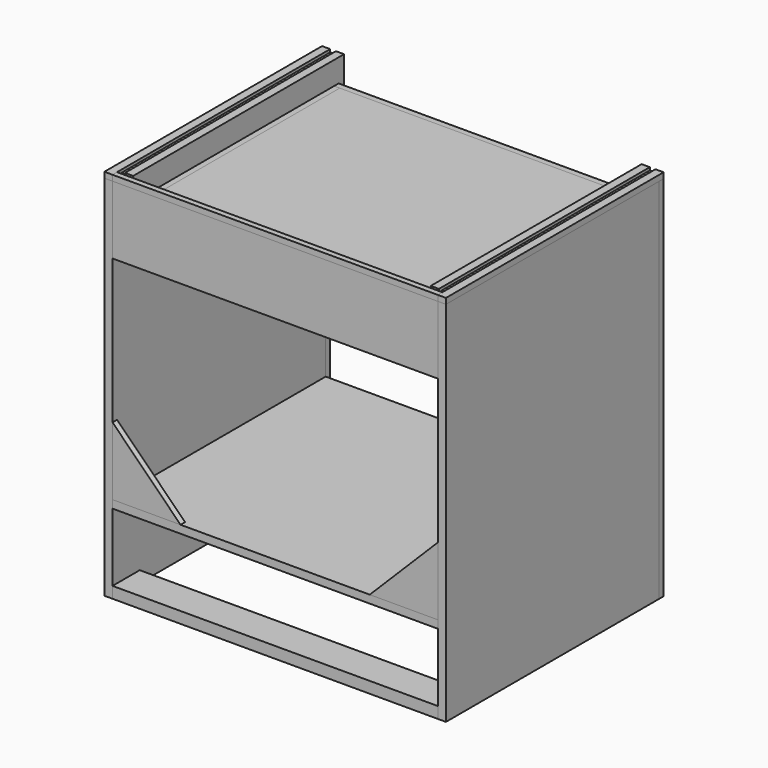
from build123d import *

# Parameters (mm, degrees)
F0_W           = 584.2
F0_H           = 208.915
F0_W_2         = 25.4
F0_W_3         = 635
F0_H_2         = 26.67
F1_DEPTH       = 18.25625
F2_DEPTH       = 4.1402
F3_DEPTH       = 18.25625
F4_DEPTH       = 18.25625
F9_DEPTH       = 54.76875
F8_W           = 12.7
F8_H           = 546.1
F10_DEPTH      = 54.76875
F12_DEPTH      = 660.401
F16_DEPTH      = 304.8
F16_DEPTH_BACK = 285.75
F15_W          = 12.7
F15_H          = 35.56
F17_DEPTH      = 304.8
F17_DEPTH_BACK = 279.4
F18_DEPTH      = 694.53225
F18_DEPTH_BACK = 34.13225
F19_W          = 18.25625
F19_H          = 12.7
F20_DEPTH      = 304.8
F19_H_2        = 823.515625
F21_DEPTH      = 304.8
F21_DEPTH_BACK = 292.1
F22_W          = 18.25625
F22_H          = 12.7
F23_DEPTH      = 823.515625
F24_W          = 76.2
F24_H          = 25.4
F25_DEPTH      = 728.6625
F24_W_2        = 596.9
F24_H_2        = 17.6944031715
F26_W          = 12.7
F26_H          = 152.4
F27_DEPTH      = 728.6625
F26_H_2        = 12.7
F28_DEPTH      = 728.6625
F30_DEPTH      = 12.7
F32_DEPTH      = 703.2625


# Not quite as in the source:
# - an extrude ends at something that could not be found from the text; its depth is read off the source's solid
# - a feature of the source that left no trace in its solid (it failed there, or was rolled back) is left out
# - a pattern or mirror of a feature is missing from the dataset's text; its kind, count and spacing are read off the source's solid


with BuildPart() as f1:
    # F0 (on Top) → F1 (new body)
    with BuildSketch(Plane.XY):
        Polygon((317.5, 241.3), (-317.5, 241.3), (-317.5, 215.9), (-292.1, 215.9), (292.1, 215.9), (317.5, 215.9), align=None)
        with Locations((0, 111.4425)):
            Rectangle(F0_W, F0_H)
        with Locations((-304.8, 111.4425)):
            Rectangle(F0_W_2, F0_H)
        with Locations((304.8, 111.4425)):
            Rectangle(F0_W_2, F0_H)
        Polygon((-292.1, 6.985), (-317.5, 6.985), (-317.5, -18.415), (317.5, -18.415), (317.5, 6.985), (292.1, 6.985), align=None)
        with Locations((0, -31.75)):
            Rectangle(F0_W_3, F0_H_2)
        Polygon((317.5, -45.085), (-317.5, -45.085), (-317.5, -70.485), (-292.1, -70.485), (292.1, -70.485), (317.5, -70.485), align=None)
        with Locations((304.8, -174.9425)):
            Rectangle(F0_W_2, F0_H)
        with Locations((0, -174.9425)):
            Rectangle(F0_W, F0_H)
        Polygon((-292.1, -279.4), (-317.5, -279.4), (-317.5, -304.8), (317.5, -304.8), (317.5, -279.4), (292.1, -279.4), align=None)
        with Locations((-304.8, -174.9425)):
            Rectangle(F0_W_2, F0_H)
    extrude(amount=F1_DEPTH)


with BuildPart() as f1_copies_1:
    # F1_copies: instance of F1
    add(f1.part.mirror(Plane(origin=(0, 0, -9.128125), x_dir=(-1, 0, 0), z_dir=(0, 0, -1))))


with BuildPart() as f1_1:
    add(f1.part)

    # F0 (on Top) → F2 (cut)
    with BuildSketch(Plane.XY):
        with Locations((0, -31.75)):
            Rectangle(F0_W_3, F0_H_2)
    extrude(amount=F2_DEPTH, mode=Mode.SUBTRACT)


with BuildPart() as f3:
    # F0 (on Top) → F3 (new body)
    with BuildSketch(Plane.XY):
        Polygon((317.5, -45.085), (-317.5, -45.085), (-317.5, -70.485), (-292.1, -70.485), (292.1, -70.485), (317.5, -70.485), align=None)
    extrude(amount=-F3_DEPTH)


with BuildPart() as f3b:
    # F0 (on Top) → F3, piece 2 (new body)
    with BuildSketch(Plane.XY):
        Polygon((-292.1, 6.985), (-317.5, 6.985), (-317.5, -18.415), (317.5, -18.415), (317.5, 6.985), (292.1, 6.985), align=None)
    extrude(amount=-F3_DEPTH)


with BuildPart() as f3c:
    # F0 (on Top) → F3, piece 3 (new body)
    with BuildSketch(Plane.XY):
        Polygon((317.5, 241.3), (-317.5, 241.3), (-317.5, 215.9), (-292.1, 215.9), (292.1, 215.9), (317.5, 215.9), align=None)
    extrude(amount=-F3_DEPTH)


with BuildPart() as f3d:
    # F0 (on Top) → F3, piece 4 (new body)
    with BuildSketch(Plane.XY):
        Polygon((-292.1, -279.4), (-317.5, -279.4), (-317.5, -304.8), (317.5, -304.8), (317.5, -279.4), (292.1, -279.4), align=None)
    extrude(amount=-F3_DEPTH)


with BuildPart() as f4:
    # F0 (on Top) → F4 (new body)
    with BuildSketch(Plane.XY):
        with Locations((304.8, -174.9425)):
            Rectangle(F0_W_2, F0_H)
    extrude(amount=-F4_DEPTH)


with BuildPart() as f4b:
    # F0 (on Top) → F4, piece 2 (new body)
    with BuildSketch(Plane.XY):
        with Locations((304.8, 111.4425)):
            Rectangle(F0_W_2, F0_H)
    extrude(amount=-F4_DEPTH)


with BuildPart() as f4c:
    # F0 (on Top) → F4, piece 3 (new body)
    with BuildSketch(Plane.XY):
        with Locations((-304.8, 111.4425)):
            Rectangle(F0_W_2, F0_H)
    extrude(amount=-F4_DEPTH)


with BuildPart() as f4d:
    # F0 (on Top) → F4, piece 4 (new body)
    with BuildSketch(Plane.XY):
        with Locations((-304.8, -174.9425)):
            Rectangle(F0_W_2, F0_H)
    extrude(amount=-F4_DEPTH)


with BuildPart() as f9:
    # F8 (on face) → F9 (new body, through all)
    with BuildSketch(Plane.XY.offset(18.25625)):
        Polygon((317.5, -304.8), (-317.5, -304.8), (-330.2, -304.8), (-330.2, -317.5), (330.2, -317.5), (330.2, -304.8), align=None)
    extrude(amount=-F9_DEPTH)


with BuildPart() as f9b:
    # F8 (on face) → F9, piece 2 (new body, through all)
    with BuildSketch(Plane.XY.offset(18.25625)):
        Polygon((-330.2, 241.3), (-317.5, 241.3), (317.5, 241.3), (330.2, 241.3), (330.2, 254), (-330.2, 254), align=None)
    extrude(amount=-F9_DEPTH)


with BuildPart() as f10:
    # F8 (on face) → F10 (new body, through all)
    with BuildSketch(Plane.XY.offset(18.25625)):
        with Locations((323.85, -31.75)):
            Rectangle(F8_W, F8_H)
    extrude(amount=-F10_DEPTH)


with BuildPart() as f10b:
    # F8 (on face) → F10, piece 2 (new body, through all)
    with BuildSketch(Plane.XY.offset(18.25625)):
        with Locations((-323.85, -31.75)):
            Rectangle(F8_W, F8_H)
    extrude(amount=-F10_DEPTH)


with BuildPart() as f12_tool:
    # F11 (on face) → F12 (new body, through all)
    with BuildSketch(Plane(origin=(-330.2, 0, 0), x_dir=(0, -1, 0), z_dir=(-1, 0, 0))):
        Polygon((18.415, -18.25625), (18.415, -22.39645), (45.085, -22.39645), (45.085, -18.25625), (45.085, 0), (45.085, 4.1402), (18.415, 4.1402), (18.415, 0), align=None)
    extrude(amount=-F12_DEPTH)


with BuildPart() as f1_copies_1_1:
    add(f1_copies_1.part)

    # F12: cut by f12_tool
    add(f12_tool.part, mode=Mode.SUBTRACT)


with BuildPart() as f10_1:
    add(f10.part)

    # F12: cut by f12_tool
    add(f12_tool.part, mode=Mode.SUBTRACT)


with BuildPart() as f10b_1:
    add(f10b.part)

    # F12: cut by f12_tool
    add(f12_tool.part, mode=Mode.SUBTRACT)


with BuildPart() as f16:
    # F15 (on face) → F16 (new body, two sides)
    with BuildSketch(Plane.XZ.offset(31.75)) as f16_sk:
        Polygon((-333.375, -85.328125), (-333.375, 67.071875), (-351.63125, 67.071875), (-351.63125, 60.721875), (-351.63125, 25.161875), (-351.63125, -43.418125), (-351.63125, -78.978125), (-351.63125, -85.328125), align=None)
    extrude(amount=-F16_DEPTH)
    extrude(f16_sk.sketch, amount=F16_DEPTH_BACK)


with BuildPart() as f16b:
    # F15 (on face) → F16, piece 2 (new body, two sides)
    with BuildSketch(Plane.XZ.offset(31.75)) as f16_2_sk:
        Polygon((351.63125, 67.071875), (333.375, 67.071875), (333.375, -85.328125), (351.63125, -85.328125), (351.63125, -78.978125), (351.63125, -43.418125), (351.63125, 25.161875), (351.63125, 60.721875), align=None)
    extrude(amount=-F16_DEPTH)
    extrude(f16_2_sk.sketch, amount=F16_DEPTH_BACK)


with BuildPart() as f17:
    # F15 (on face) → F17 (new body, two sides)
    with BuildSketch(Plane.XZ.offset(31.75)) as f17_sk:
        with Locations((-357.98125, 42.941875)):
            Rectangle(F15_W, F15_H)
    extrude(amount=-F17_DEPTH)
    extrude(f17_sk.sketch, amount=F17_DEPTH_BACK)


with BuildPart() as f17b:
    # F15 (on face) → F17, piece 2 (new body, two sides)
    with BuildSketch(Plane.XZ.offset(31.75)) as f17_2_sk:
        with Locations((-357.98125, -61.198125)):
            Rectangle(F15_W, F15_H)
    extrude(amount=-F17_DEPTH)
    extrude(f17_2_sk.sketch, amount=F17_DEPTH_BACK)


with BuildPart() as f17c:
    # F15 (on face) → F17, piece 3 (new body, two sides)
    with BuildSketch(Plane.XZ.offset(31.75)) as f17_3_sk:
        with Locations((357.98125, 42.941875)):
            Rectangle(F15_W, F15_H)
    extrude(amount=-F17_DEPTH)
    extrude(f17_3_sk.sketch, amount=F17_DEPTH_BACK)


with BuildPart() as f17d:
    # F15 (on face) → F17, piece 4 (new body, two sides)
    with BuildSketch(Plane.XZ.offset(31.75)) as f17_4_sk:
        with Locations((357.98125, -61.198125)):
            Rectangle(F15_W, F15_H)
    extrude(amount=-F17_DEPTH)
    extrude(f17_4_sk.sketch, amount=F17_DEPTH_BACK)


with BuildPart() as f18_tool:
    # F11 (on face) → F18 (new body, two sides)
    with BuildSketch(Plane(origin=(-330.2, 0, 0), x_dir=(0, -1, 0), z_dir=(-1, 0, 0))) as f18_sk:
        Polygon((18.415, -18.25625), (18.415, -22.39645), (45.085, -22.39645), (45.085, -18.25625), (45.085, 0), (45.085, 4.1402), (18.415, 4.1402), (18.415, 0), align=None)
    extrude(amount=-F18_DEPTH)
    extrude(f18_sk.sketch, amount=F18_DEPTH_BACK)


with BuildPart() as f16_1:
    add(f16.part)

    # F18: cut by f18_tool
    add(f18_tool.part, mode=Mode.SUBTRACT)


with BuildPart() as f16b_1:
    add(f16b.part)

    # F18: cut by f18_tool
    add(f18_tool.part, mode=Mode.SUBTRACT)


with BuildPart() as f20:
    # F19 (on face) → F20 (new body, symmetric)
    with BuildSketch(Plane.XZ.offset(31.75)):
        with Locations((-373.459375, 60.721875)):
            Rectangle(F19_W, F19_H)
    extrude(amount=F20_DEPTH, both=True)


with BuildPart() as f20b:
    # F19 (on face) → F20, piece 2 (new body, symmetric)
    with BuildSketch(Plane.XZ.offset(31.75)):
        with Locations((373.459375, 60.721875)):
            Rectangle(F19_W, F19_H)
    extrude(amount=F20_DEPTH, both=True)


with BuildPart() as f21:
    # F19 (on face) → F21 (new body, two sides)
    with BuildSketch(Plane.XZ.offset(31.75)) as f21_sk:
        with Locations((-373.459375, -357.3859375)):
            Rectangle(F19_W, F19_H_2)
    extrude(amount=F21_DEPTH)
    extrude(f21_sk.sketch, amount=-F21_DEPTH_BACK)


with BuildPart() as f21b:
    # F19 (on face) → F21, piece 2 (new body, two sides)
    with BuildSketch(Plane.XZ.offset(31.75)) as f21_2_sk:
        with Locations((373.459375, -357.3859375)):
            Rectangle(F19_W, F19_H_2)
    extrude(amount=F21_DEPTH)
    extrude(f21_2_sk.sketch, amount=-F21_DEPTH_BACK)


with BuildPart() as f23:
    # F22 (on face) → F23 (new body, through all)
    with BuildSketch(Plane(origin=(0, 0, 54.371875), x_dir=(1, 0, 0), z_dir=(0, 0, -1))):
        with Locations((-373.459375, -266.7)):
            Rectangle(F22_W, F22_H)
    extrude(amount=F23_DEPTH)


with BuildPart() as f23b:
    # F22 (on face) → F23, piece 2 (new body, through all)
    with BuildSketch(Plane(origin=(0, 0, 54.371875), x_dir=(1, 0, 0), z_dir=(0, 0, -1))):
        with Locations((373.459375, -266.7)):
            Rectangle(F22_W, F22_H)
    extrude(amount=F23_DEPTH)


with BuildPart() as f25:
    # F24 (on face) → F25 (new body, through all)
    with BuildSketch(Plane(origin=(364.33125, 0, 0), x_dir=(0, -1, 0), z_dir=(-1, 0, 0))):
        with Locations((-222.25, -756.44375)):
            Rectangle(F24_W, F24_H)
    extrude(amount=F25_DEPTH)


with BuildPart() as f25b:
    # F24 (on face) → F25, piece 2 (new body, through all)
    with BuildSketch(Plane(origin=(364.33125, 0, 0), x_dir=(0, -1, 0), z_dir=(-1, 0, 0))):
        with Locations((298.45, -756.44375)):
            Rectangle(F24_W, F24_H)
    extrude(amount=F25_DEPTH)


with BuildPart() as f25c:
    # F24 (on face) → F25, piece 3 (new body, through all)
    with BuildSketch(Plane(origin=(364.33125, 0, 0), x_dir=(0, -1, 0), z_dir=(-1, 0, 0))):
        with Locations((38.1, -582.4965484142)):
            Rectangle(F24_W_2, F24_H_2)
    extrude(amount=F25_DEPTH)


with BuildPart() as f27:
    # F26 (on face) → F27 (new body, through all)
    with BuildSketch(Plane.YZ.offset(-364.33125)):
        with Locations((-330.2, -21.828125)):
            Rectangle(F26_W, F26_H)
    extrude(amount=F27_DEPTH)


with BuildPart() as f28:
    # F26 (on face) → F28 (new body, through all)
    with BuildSketch(Plane.YZ.offset(-364.33125)):
        with Locations((-330.2, 60.721875)):
            Rectangle(F26_W, F26_H_2)
    extrude(amount=F28_DEPTH)


with BuildPart() as f30:
    # F29 (on face) → F30 (new body)
    with BuildSketch(Plane.XZ.offset(336.55)):
        Polygon((-364.33125, -421.2493468285), (-364.33125, -573.6493468285), (-211.93125, -573.6493468285), align=None)
    extrude(amount=-F30_DEPTH)


with BuildPart() as f30b:
    # F29 (on face) → F30, piece 2 (new body)
    with BuildSketch(Plane.XZ.offset(336.55)):
        Polygon((211.93125, -573.6493468285), (364.33125, -573.6493468285), (364.33125, -421.2493468285), align=None)
    extrude(amount=-F30_DEPTH)


with BuildPart() as f32:
    # F31 (on face) → F32 (new body, through all)
    with BuildSketch(Plane(origin=(-351.63125, 0, 0), x_dir=(0, -1, 0), z_dir=(-1, 0, 0))):
        with BuildLine():
            ThreePointArc((31.75, -22.39645), (41.1321225825, -18.5102475825), (45.018325, -9.128125))
            ThreePointArc((45.018325, -9.128125), (41.1321225825, 0.2539975825), (31.75, 4.1402))
            ThreePointArc((31.75, 4.1402), (18.481675, -9.128125), (31.75, -22.39645))
        make_face()
    extrude(amount=-F32_DEPTH)


solid = Compound([f1_1.part, f3.part, f3b.part, f3c.part, f3d.part, f4.part, f4b.part, f4c.part, f4d.part, f9.part, f9b.part, f1_copies_1_1.part, f10_1.part, f10b_1.part, f17.part, f17b.part, f17c.part, f17d.part, f16_1.part, f16b_1.part, f20.part, f20b.part, f21.part, f21b.part, f23.part, f23b.part, f25.part, f25b.part, f25c.part, f27.part, f28.part, f30.part, f30b.part, f32.part])
